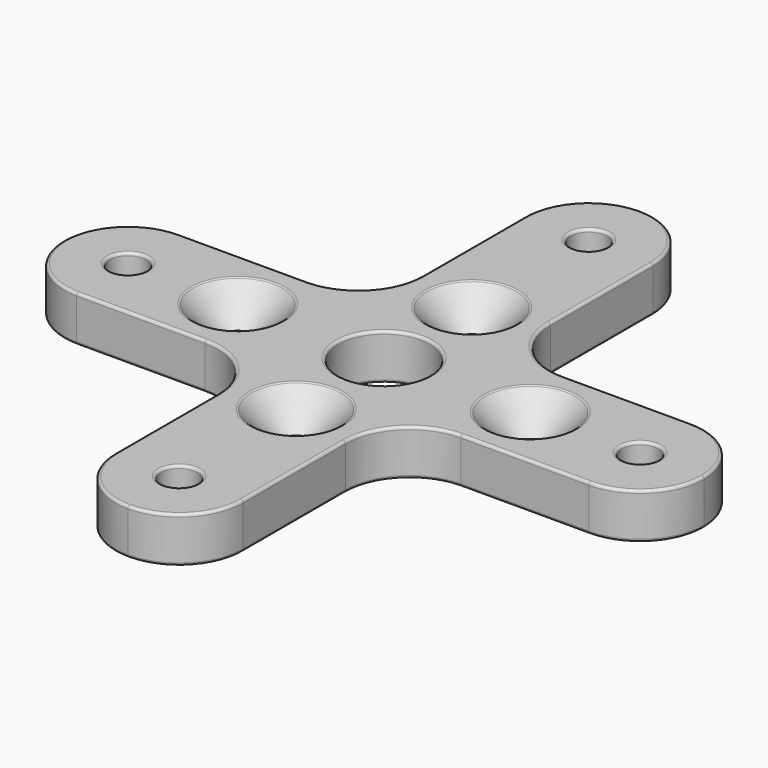
from build123d import *

# Parameters (mm, degrees)
F0_R     = 1
F0_R_2   = 0.8
F0_R_3   = 2.5
F1_DEPTH = 2.5
F2_R     = 3.49999
F3_SIZE  = 1.7
F4_R     = 0.15


# Not quite as in the source:
# - a fillet or chamfer is up to 0.001 mm smaller than in the source, because OpenCascade refuses the exact size


with BuildPart() as f1:
    # F0 (on Top) → F1 (new body)
    with BuildSketch(Plane.XY):
        Polygon((-24.8403990492, -37.8702705037), (-17.8403990492, -37.8702705037), (-17.8403990492, -23.8702705037), (-3.8403990492, -23.8702705037), (-3.8403990492, -16.8702705037), (-17.8403990492, -16.8702705037), (-17.8403990492, -2.8702705037), (-24.8403990492, -2.8702705037), (-24.8403990492, -16.8702705037), (-38.8403990492, -16.8702705037), (-38.8403990492, -23.8702705037), (-24.8403990492, -23.8702705037), align=None)
        with Locations((-21.3403990492, -34.3702705037)):
            Circle(F0_R, mode=Mode.SUBTRACT)
        with Locations((-21.3403990492, -26.3702705037)):
            Circle(F0_R_2, mode=Mode.SUBTRACT)
        with Locations((-35.3403990492, -20.3702705037)):
            Circle(F0_R, mode=Mode.SUBTRACT)
        with Locations((-29.3403990492, -20.3702705037)):
            Circle(F0_R_2, mode=Mode.SUBTRACT)
        with Locations((-21.3403990492, -14.3702705037)):
            Circle(F0_R_2, mode=Mode.SUBTRACT)
        with Locations((-21.3403990492, -6.3702705037)):
            Circle(F0_R, mode=Mode.SUBTRACT)
        with Locations((-21.3403990492, -20.3702705037)):
            Circle(F0_R_3, mode=Mode.SUBTRACT)
        with Locations((-13.3403990492, -20.3702705037)):
            Circle(F0_R_2, mode=Mode.SUBTRACT)
        with Locations((-7.3403990492, -20.3702705037)):
            Circle(F0_R, mode=Mode.SUBTRACT)
    extrude(amount=F1_DEPTH)

    # F2 (radius 3.5 in the source; OpenCascade refuses exactly that, so slightly less here)
    f2_edges = [f1.edges().sort_by_distance(p)[0] for p in [
        (-24.840399, -2.870271, 1.25),
        (-17.840399, -2.870271, 1.25),
        (-3.840399, -16.870271, 1.25),
        (-3.840399, -23.870271, 1.25),
        (-17.840399, -37.870271, 1.25),
        (-24.840399, -37.870271, 1.25),
        (-38.840399, -23.870271, 1.25),
        (-38.840399, -16.870271, 1.25),
        (-24.840399, -23.870271, 1.25),
        (-17.840399, -23.870271, 1.25),
        (-17.840399, -16.870271, 1.25),
        (-24.840399, -16.870271, 1.25),
    ]]
    fillet(f2_edges, radius=F2_R)

    # F3
    f3_edges = [f1.edges().sort_by_distance(p)[0] for p in [
        (-22.140399, -14.370271, 2.5),
        (-14.140399, -20.370271, 2.5),
        (-22.140399, -26.370271, 2.5),
        (-30.140399, -20.370271, 2.5),
    ]]
    chamfer(f3_edges, length=F3_SIZE)

    # F4
    f4_edges = [f1.edges().sort_by_distance(p)[0] for p in [
        (-23.840399, -14.370271, 2.5),
        (-31.840399, -23.870271, 2.5),
        (-37.815276, -22.845147, 2.5),
        (-25.865522, -24.895394, 2.5),
        (-38.840399, -20.370271, 2.5),
        (-24.840399, -30.870271, 2.5),
        (-37.815276, -17.895394, 2.5),
        (-23.815276, -36.845147, 2.5),
        (-31.840399, -16.870271, 2.5),
        (-21.340399, -37.870271, 2.5),
        (-25.865522, -15.845147, 2.5),
        (-18.865522, -36.845147, 2.5),
        (-24.840399, -9.870271, 2.5),
        (-17.840399, -30.870271, 2.5),
        (-23.815276, -3.895394, 2.5),
        (-16.815276, -24.895394, 2.5),
        (-21.340399, -2.870271, 2.5),
        (-10.840399, -23.870271, 2.5),
        (-18.865522, -3.895394, 2.5),
        (-4.865522, -22.845147, 2.5),
        (-17.840399, -9.870271, 2.5),
        (-3.840399, -20.370271, 2.5),
        (-16.815276, -15.845147, 2.5),
        (-4.865522, -17.895394, 2.5),
        (-10.840399, -16.870271, 2.5),
        (-22.340399, -34.370271, 2.5),
        (-36.340399, -20.370271, 2.5),
        (-22.340399, -6.370271, 2.5),
        (-23.840399, -20.370271, 2.5),
        (-8.340399, -20.370271, 2.5),
        (-15.840399, -20.370271, 2.5),
        (-23.840399, -26.370271, 2.5),
        (-31.840399, -20.370271, 2.5),
        (-31.840399, -23.870271, 0),
        (-37.815276, -22.845147, 0),
        (-25.865522, -24.895394, 0),
        (-38.840399, -20.370271, 0),
        (-24.840399, -30.870271, 0),
        (-37.815276, -17.895394, 0),
        (-23.815276, -36.845147, 0),
        (-31.840399, -16.870271, 0),
        (-21.340399, -37.870271, 0),
        (-25.865522, -15.845147, 0),
        (-18.865522, -36.845147, 0),
        (-24.840399, -9.870271, 0),
        (-17.840399, -30.870271, 0),
        (-23.815276, -3.895394, 0),
        (-16.815276, -24.895394, 0),
        (-21.340399, -2.870271, 0),
        (-10.840399, -23.870271, 0),
        (-18.865522, -3.895394, 0),
        (-4.865522, -22.845147, 0),
        (-17.840399, -9.870271, 0),
        (-3.840399, -20.370271, 0),
        (-16.815276, -15.845147, 0),
        (-4.865522, -17.895394, 0),
        (-10.840399, -16.870271, 0),
        (-22.340399, -34.370271, 0),
        (-22.140399, -26.370271, 0),
        (-36.340399, -20.370271, 0),
        (-30.140399, -20.370271, 0),
        (-22.140399, -14.370271, 0),
        (-22.340399, -6.370271, 0),
        (-23.840399, -20.370271, 0),
        (-14.140399, -20.370271, 0),
        (-8.340399, -20.370271, 0),
    ]]
    fillet(f4_edges, radius=F4_R)


solid = f1.part
